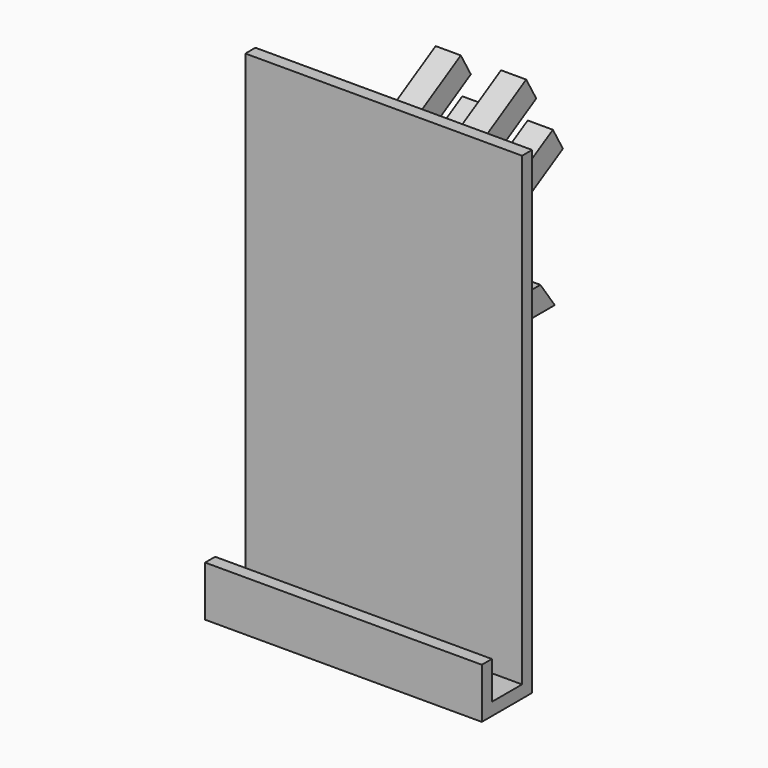
from build123d import *

# Parameters (mm, degrees)
F0_W     = 15
F0_H     = 5
F1_DEPTH = 110
F2_W     = 8
F2_H     = 98.8297045976
F2_W_2   = 37
F2_H_2   = 91.1702954024
F2_W_3   = 10
F3_DEPTH = 100


# Not quite as in the source:
# - a feature of the source that left no trace in its solid (it failed there, or was rolled back) is left out


with BuildPart() as f1:
    # F0 (on Right) → F1 (new body)
    with BuildSketch(Plane.YZ):
        Polygon((30.635715595, 45.1382968587), (0, 27.4507582131), (0, 15.9037528294), (36.4732290688, 36.9615814504), align=None)
        Polygon((56.5512701892, 60.1006492799), (30.635715595, 45.1382968587), (36.4732290688, 36.9615814504), (61.5512701892, 51.4403952421), align=None)
        Polygon((15.1663048896, 66.8065926908), (0, 58.0503224802), (0, 46.5033170964), (21.0038183633, 58.6298772825), align=None)
        Polygon((43.3012701892, 83.0503224802), (15.1663048896, 66.8065926908), (21.0038183633, 58.6298772825), (48.3012701892, 74.3900684424), align=None)
        Polygon((-20, -101.9496775198), (-20, -96.9496775198), (-20, -81.9496775198), (-25, -81.9496775198), (-25, -101.9496775198), align=None)
        with Locations((-12.5, -99.4496775198)):
            Rectangle(F0_W, F0_H)
        Polygon((0, 88.0503224802), (-5, 88.0503224802), (-5, -96.9496775198), (-5, -101.9496775198), (0, -101.9496775198), (0, -10), (0, 0), (0, 15.9037528294), (0, 27.4507582131), (0, 46.5033170964), (0, 58.0503224802), align=None)
        Polygon((0, 0), (0, -10), (70, -10), (62.860808794, 0), align=None)
    extrude(amount=F1_DEPTH)

    # F2 (on Front) → F3 (cut)
    with BuildSketch(Plane.XZ):
        with Locations((51, 64.6969747171)):
            Rectangle(F2_W, F2_H)
        with Locations((59, 64.6969747171)):
            Rectangle(F2_W, F2_H)
        with Locations((91.5, -30.3030252829)):
            Rectangle(F2_W_2, F2_H_2)
        with Locations((18.5, -30.3030252829)):
            Rectangle(F2_W_2, F2_H_2)
        with Locations((42, -30.3030252829)):
            Rectangle(F2_W_3, F2_H_2)
        with Locations((68, -30.3030252829)):
            Rectangle(F2_W_3, F2_H_2)
        with Locations((91.5, 64.6969747171)):
            Rectangle(F2_W_2, F2_H)
        with Locations((18.5, 64.6969747171)):
            Rectangle(F2_W_2, F2_H)
    extrude(amount=-F3_DEPTH, mode=Mode.SUBTRACT)


solid = f1.part
